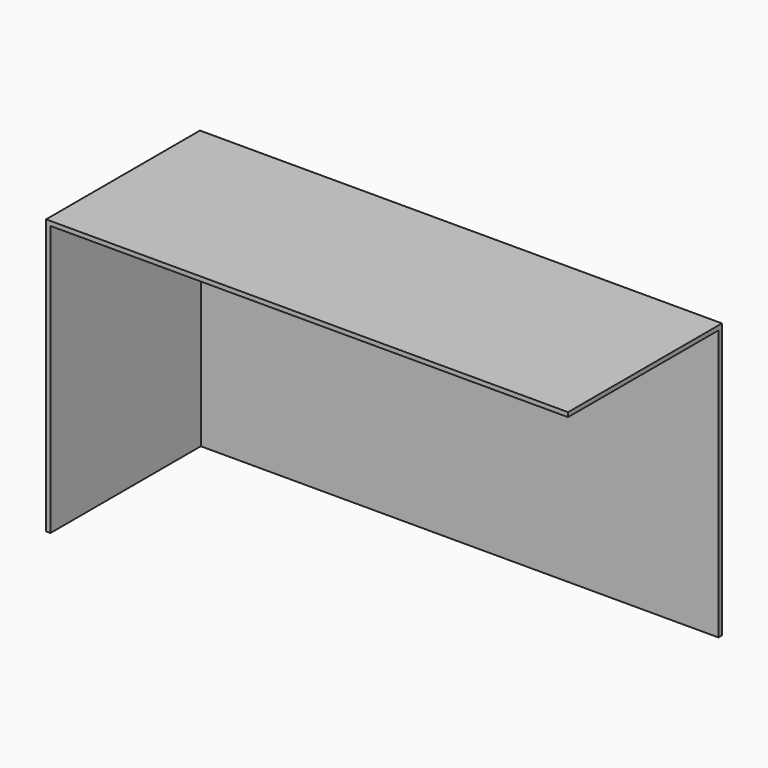
from build123d import *

# Parameters (mm, degrees)
F0_W     = 1900
F0_H     = 700
F1_DEPTH = 1000
F2_T     = -16


# Not quite as in the source:
# - a feature names something its author has since deleted; it is built from what else it names


with BuildPart() as f1:
    # F0 (on Top) → F1 (new body)
    with BuildSketch(Plane.XY):
        with Locations((-950, -350)):
            Rectangle(F0_W, F0_H)
    extrude(amount=F1_DEPTH)

    # F2
    f2_openings = [f1.faces().sort_by_distance(p)[0] for p in [
        (-950, -350, 0),
        (-950, -700, 500),
        (0, -350, 500),
    ]]
    offset(amount=F2_T, openings=f2_openings)


solid = f1.part
